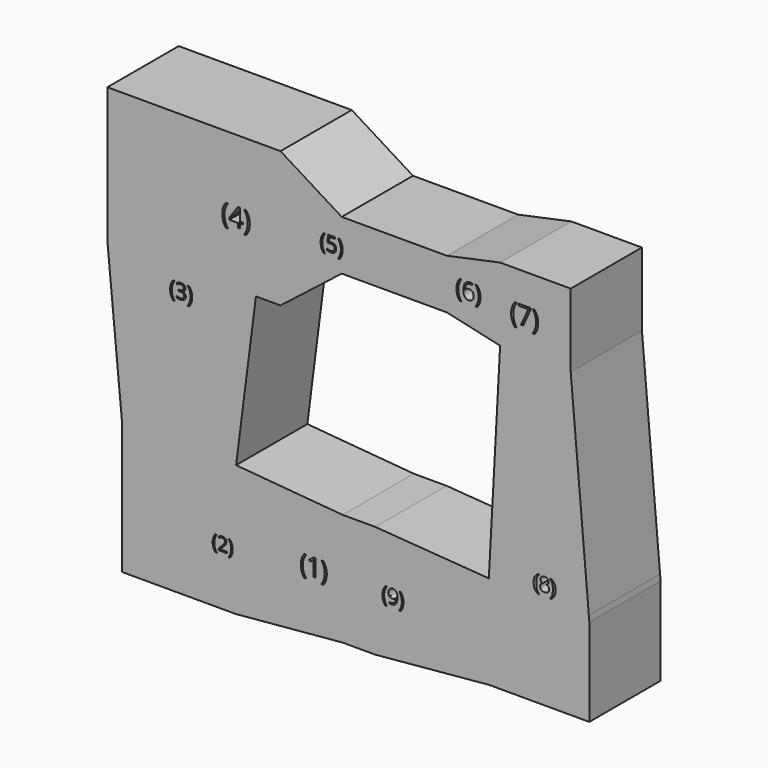
from build123d import *

# Parameters (mm, degrees)
F0_W     = 7.0054735818
F0_H     = 3.606621176
F0_H_2   = 2.8473325074
F0_H_3   = 3.0371509492
F0_H_4   = 3.4167952836
F0_H_5   = 3.4167990088
F0_H_6   = 3.0424887748
F0_H_7   = 3.4114611833
F0_H_8   = 3.2269731164
F0_H_9   = 2.668182266
F0_W_2   = 20.1211348176
F0_H_10  = 20.8804234862
F0_W_3   = 9.3167445157
F0_H_11  = 32.0711014792
F1_DEPTH = 12.7


with BuildPart() as f1:
    # F0 (on Front) → F1 (new body, symmetric)
    with BuildSketch(Plane.XZ):
        Polygon((-30.1637667992, 35.9712801874), (-72.5167479517, 35.9712801874), (-68.335942924, -8.2572624087), (-35.8229727803, -8.2572624087), align=None)
        with BuildLine():
            add(Edge.make_bspline(
                [(-54.4081610007, 28.3956593022), (-54.6265717389, 29.0386568902), (-54.6265717389, 29.777265818)],
                knots=[0, 0, 0, 1, 1, 1], degree=2))
            add(Edge.make_bspline(
                [(-54.6265717389, 29.777265818), (-54.6265717389, 30.5276562378), (-54.4068015978, 31.1819821836)],
                knots=[0, 0, 0, 1, 1, 1], degree=2))
            add(Edge.make_bspline(
                [(-54.4068015978, 31.1819821836), (-54.1870314567, 31.8363081294), (-53.7737729646, 32.3293182604)],
                knots=[0, 0, 0, 1, 1, 1], degree=2))
            Line((-53.7737729646, 32.3293182604), (-53.3152010414, 32.3293182604))
            add(Edge.make_bspline(
                [(-53.3152010414, 32.3293182604), (-53.7230219217, 31.7828382807), (-53.9282917649, 31.1285123349)],
                knots=[0, 0, 0, 1, 1, 1], degree=2))
            add(Edge.make_bspline(
                [(-53.9282917649, 31.1285123349), (-54.133561608, 30.4741863891), (-54.133561608, 29.7827034297)],
                knots=[0, 0, 0, 1, 1, 1], degree=2))
            add(Edge.make_bspline(
                [(-54.133561608, 29.7827034297), (-54.133561608, 29.1030019624), (-53.9237604217, 28.4545667627)],
                knots=[0, 0, 0, 1, 1, 1], degree=2))
            add(Edge.make_bspline(
                [(-53.9237604217, 28.4545667627), (-53.7139592355, 27.8061315629), (-53.3206386531, 27.2705268067)],
                knots=[0, 0, 0, 1, 1, 1], degree=2))
            Line((-53.3206386531, 27.2705268067), (-53.7737729646, 27.2705268067))
            add(Edge.make_bspline(
                [(-53.7737729646, 27.2705268067), (-54.1897502626, 27.7526617142), (-54.4081610007, 28.3956593022)],
                knots=[0, 0, 0, 1, 1, 1], degree=2))
        make_face(mode=Mode.SUBTRACT)
        with BuildLine():
            add(Edge.make_bspline(
                [(-50.6272083055, 32.1122669251), (-50.2927951836, 31.8363081294), (-50.2927951836, 31.3550794906)],
                knots=[0, 0, 0, 1, 1, 1], degree=2))
            add(Edge.make_bspline(
                [(-50.2927951836, 31.3550794906), (-50.2927951836, 30.9581338337), (-50.5152841306, 30.7061911565)],
                knots=[0, 0, 0, 1, 1, 1], degree=2))
            add(Edge.make_bspline(
                [(-50.5152841306, 30.7061911565), (-50.7377730775, 30.4542484793), (-51.1455939579, 30.3690592288)],
                knots=[0, 0, 0, 1, 1, 1], degree=2))
            Line((-51.1455939579, 30.3690592288), (-51.1455939579, 30.3464025132))
            add(Edge.make_bspline(
                [(-51.1455939579, 30.3464025132), (-50.6471462152, 30.2847762468), (-50.4065318958, 30.0296616295)],
                knots=[0, 0, 0, 1, 1, 1], degree=2))
            add(Edge.make_bspline(
                [(-50.4065318958, 30.0296616295), (-50.1659175764, 29.7745470121), (-50.1659175764, 29.36128852)],
                knots=[0, 0, 0, 1, 1, 1], degree=2))
            add(Edge.make_bspline(
                [(-50.1659175764, 29.36128852), (-50.1659175764, 28.7694951092), (-50.5764572627, 28.4504885539)],
                knots=[0, 0, 0, 1, 1, 1], degree=2))
            add(Edge.make_bspline(
                [(-50.5764572627, 28.4504885539), (-50.9869969489, 28.1314819986), (-51.7428249805, 28.1314819986)],
                knots=[0, 0, 0, 1, 1, 1], degree=2))
            add(Edge.make_bspline(
                [(-51.7428249805, 28.1314819986), (-52.0718004906, 28.1314819986), (-52.3450404805, 28.1813267728)],
                knots=[0, 0, 0, 1, 1, 1], degree=2))
            add(Edge.make_bspline(
                [(-52.3450404805, 28.1813267728), (-52.6182804703, 28.2311715471), (-52.8756607592, 28.3553303485)],
                knots=[0, 0, 0, 1, 1, 1], degree=2))
            Line((-52.8756607592, 28.3553303485), (-52.8756607592, 28.8030270482))
            add(Edge.make_bspline(
                [(-52.8756607592, 28.8030270482), (-52.6064989782, 28.6698055606), (-52.3019927209, 28.600476011)],
                knots=[0, 0, 0, 1, 1, 1], degree=2))
            add(Edge.make_bspline(
                [(-52.3019927209, 28.600476011), (-51.9974864635, 28.5311464613), (-51.7256058766, 28.5311464613)],
                knots=[0, 0, 0, 1, 1, 1], degree=2))
            add(Edge.make_bspline(
                [(-51.7256058766, 28.5311464613), (-50.652583827, 28.5311464613), (-50.652583827, 29.3721637435)],
                knots=[0, 0, 0, 1, 1, 1], degree=2))
            add(Edge.make_bspline(
                [(-50.652583827, 29.3721637435), (-50.652583827, 30.1261792378), (-51.8361706486, 30.1261792378)],
                knots=[0, 0, 0, 1, 1, 1], degree=2))
            Line((-51.8361706486, 30.1261792378), (-52.243991529, 30.1261792378))
            Line((-52.243991529, 30.1261792378), (-52.243991529, 30.5303750437))
            Line((-52.243991529, 30.5303750437), (-51.8307330369, 30.5303750437))
            add(Edge.make_bspline(
                [(-51.8307330369, 30.5303750437), (-51.3467855922, 30.5303750437), (-51.0635766475, 30.7442544387)],
                knots=[0, 0, 0, 1, 1, 1], degree=2))
            add(Edge.make_bspline(
                [(-51.0635766475, 30.7442544387), (-50.7803677028, 30.9581338337), (-50.7803677028, 31.3378603868)],
                knots=[0, 0, 0, 1, 1, 1], degree=2))
            add(Edge.make_bspline(
                [(-50.7803677028, 31.3378603868), (-50.7803677028, 31.6405541069), (-50.9883563518, 31.8136514139)],
                knots=[0, 0, 0, 1, 1, 1], degree=2))
            add(Edge.make_bspline(
                [(-50.9883563518, 31.8136514139), (-51.1963450008, 31.9867487209), (-51.5534148383, 31.9867487209)],
                knots=[0, 0, 0, 1, 1, 1], degree=2))
            add(Edge.make_bspline(
                [(-51.5534148383, 31.9867487209), (-51.8252954252, 31.9867487209), (-52.0659097446, 31.9128878281)],
                knots=[0, 0, 0, 1, 1, 1], degree=2))
            add(Edge.make_bspline(
                [(-52.0659097446, 31.9128878281), (-52.306524064, 31.8390269353), (-52.6155616644, 31.6405541069)],
                knots=[0, 0, 0, 1, 1, 1], degree=2))
            Line((-52.6155616644, 31.6405541069), (-52.8530040437, 31.9577481249))
            add(Edge.make_bspline(
                [(-52.8530040437, 31.9577481249), (-52.5983425606, 32.1589397592), (-52.2657419759, 32.27358274)],
                knots=[0, 0, 0, 1, 1, 1], degree=2))
            add(Edge.make_bspline(
                [(-52.2657419759, 32.27358274), (-51.9331413913, 32.3882257209), (-51.5642900617, 32.3882257209)],
                knots=[0, 0, 0, 1, 1, 1], degree=2))
            add(Edge.make_bspline(
                [(-51.5642900617, 32.3882257209), (-50.9616214274, 32.3882257209), (-50.6272083055, 32.1122669251)],
                knots=[0, 0, 0, 1, 1, 1], degree=2))
        make_face(mode=Mode.SUBTRACT)
        with BuildLine():
            add(Edge.make_bspline(
                [(-48.5600095765, 31.1779039748), (-48.3415988383, 30.5222186261), (-48.3415988383, 29.777265818)],
                knots=[0, 0, 0, 1, 1, 1], degree=2))
            add(Edge.make_bspline(
                [(-48.3415988383, 29.777265818), (-48.3415988383, 29.0323130098), (-48.5613689794, 28.3893154218)],
                knots=[0, 0, 0, 1, 1, 1], degree=2))
            add(Edge.make_bspline(
                [(-48.5613689794, 28.3893154218), (-48.7811391205, 27.7463178338), (-49.1943976126, 27.2705268067)],
                knots=[0, 0, 0, 1, 1, 1], degree=2))
            Line((-49.1943976126, 27.2705268067), (-49.6475319241, 27.2705268067))
            add(Edge.make_bspline(
                [(-49.6475319241, 27.2705268067), (-49.2542113417, 27.803412757), (-49.0444101555, 28.4532073597)],
                knots=[0, 0, 0, 1, 1, 1], degree=2))
            add(Edge.make_bspline(
                [(-49.0444101555, 28.4532073597), (-48.8346089692, 29.1030019624), (-48.8346089692, 29.7827034297)],
                knots=[0, 0, 0, 1, 1, 1], degree=2))
            add(Edge.make_bspline(
                [(-48.8346089692, 29.7827034297), (-48.8346089692, 30.4741863891), (-49.0398788123, 31.1285123349)],
                knots=[0, 0, 0, 1, 1, 1], degree=2))
            add(Edge.make_bspline(
                [(-49.0398788123, 31.1285123349), (-49.2451486554, 31.7828382807), (-49.6529695358, 32.3293182604)],
                knots=[0, 0, 0, 1, 1, 1], degree=2))
            Line((-49.6529695358, 32.3293182604), (-49.1943976126, 32.3293182604))
            add(Edge.make_bspline(
                [(-49.1943976126, 32.3293182604), (-48.7784203146, 31.8335893236), (-48.5600095765, 31.1779039748)],
                knots=[0, 0, 0, 1, 1, 1], degree=2))
        make_face(mode=Mode.SUBTRACT)
        Polygon((-30.1637667992, 74.7056555869), (-72.5167479517, 74.7056555869), (-72.5167479517, 35.9712801874), (-30.1637667992, 35.9712801874), (-30.1637667992, 39.5779013634), (-30.1637667992, 42.4252338707), (-30.1637667992, 45.46238482), (-30.1637667992, 48.8791801035), (-30.1637667992, 52.2959791124), (-30.1637667992, 55.3384678871), (-30.1637667992, 58.7499290705), (-30.1637667992, 62.1667280793), (-30.1637667992, 65.3937011957), (-30.1637667992, 68.8105002046), (-30.1637667992, 72.037473321), align=None)
        with BuildLine():
            add(Edge.make_bspline(
                [(-39.489436089, 51.7955468905), (-39.7624492438, 52.5992930868), (-39.7624492438, 53.5225533406)],
                knots=[0, 0, 0, 1, 1, 1], degree=2))
            add(Edge.make_bspline(
                [(-39.7624492438, 53.5225533406), (-39.7624492438, 54.460540445), (-39.487736837, 55.2784470747)],
                knots=[0, 0, 0, 1, 1, 1], degree=2))
            add(Edge.make_bspline(
                [(-39.487736837, 55.2784470747), (-39.2130244303, 56.0963537044), (-38.696451822, 56.7126157633)],
                knots=[0, 0, 0, 1, 1, 1], degree=2))
            Line((-38.696451822, 56.7126157633), (-38.1232374805, 56.7126157633))
            add(Edge.make_bspline(
                [(-38.1232374805, 56.7126157633), (-38.6330130807, 56.029516459), (-38.8896001328, 55.2116098293)],
                knots=[0, 0, 0, 1, 1, 1], degree=2))
            add(Edge.make_bspline(
                [(-38.8896001328, 55.2116098293), (-39.1461871849, 54.3937031996), (-39.1461871849, 53.5293503486)],
                knots=[0, 0, 0, 1, 1, 1], degree=2))
            add(Edge.make_bspline(
                [(-39.1461871849, 53.5293503486), (-39.1461871849, 52.6797243482), (-38.8839359594, 51.8691811439)],
                knots=[0, 0, 0, 1, 1, 1], degree=2))
            add(Edge.make_bspline(
                [(-38.8839359594, 51.8691811439), (-38.621684734, 51.0586379395), (-38.1300344885, 50.3891326512)],
                knots=[0, 0, 0, 1, 1, 1], degree=2))
            Line((-38.1300344885, 50.3891326512), (-38.696451822, 50.3891326512))
            add(Edge.make_bspline(
                [(-38.696451822, 50.3891326512), (-39.2164229343, 50.9918006941), (-39.489436089, 51.7955468905)],
                knots=[0, 0, 0, 1, 1, 1], degree=2))
        make_face(mode=Mode.SUBTRACT)
        Polygon((-33.9068268493, 53.2608685325), (-33.9068268493, 52.7261705696), (-34.6748887536, 52.7261705696), (-34.6748887536, 51.536694169), (-35.2379075832, 51.536694169), (-35.2379075832, 52.7261705696), (-37.7550662136, 52.7261705696), (-37.7550662136, 53.2393446738), (-35.2979478206, 56.74093663), (-34.6748887536, 56.74093663), (-34.6748887536, 53.2608685325), align=None, mode=Mode.SUBTRACT)
        with BuildLine():
            add(Edge.make_bspline(
                [(-32.1792539819, 55.2733493187), (-31.9062408271, 54.453743437), (-31.9062408271, 53.5225533406)],
                knots=[0, 0, 0, 1, 1, 1], degree=2))
            add(Edge.make_bspline(
                [(-31.9062408271, 53.5225533406), (-31.9062408271, 52.5913632442), (-32.1809532339, 51.7876170478)],
                knots=[0, 0, 0, 1, 1, 1], degree=2))
            add(Edge.make_bspline(
                [(-32.1809532339, 51.7876170478), (-32.4556656407, 50.9838708515), (-32.9722382489, 50.3891326512)],
                knots=[0, 0, 0, 1, 1, 1], degree=2))
            Line((-32.9722382489, 50.3891326512), (-33.5386555825, 50.3891326512))
            add(Edge.make_bspline(
                [(-33.5386555825, 50.3891326512), (-33.0470053369, 51.0552394355), (-32.7847541115, 51.8674818919)],
                knots=[0, 0, 0, 1, 1, 1], degree=2))
            add(Edge.make_bspline(
                [(-32.7847541115, 51.8674818919), (-32.522502886, 52.6797243482), (-32.522502886, 53.5293503486)],
                knots=[0, 0, 0, 1, 1, 1], degree=2))
            add(Edge.make_bspline(
                [(-32.522502886, 53.5293503486), (-32.522502886, 54.3937031996), (-32.7790899381, 55.2116098293)],
                knots=[0, 0, 0, 1, 1, 1], degree=2))
            add(Edge.make_bspline(
                [(-32.7790899381, 55.2116098293), (-33.0356769902, 56.029516459), (-33.5454525905, 56.7126157633)],
                knots=[0, 0, 0, 1, 1, 1], degree=2))
            Line((-33.5454525905, 56.7126157633), (-32.9722382489, 56.7126157633))
            add(Edge.make_bspline(
                [(-32.9722382489, 56.7126157633), (-32.4522671367, 56.0929552004), (-32.1792539819, 55.2733493187)],
                knots=[0, 0, 0, 1, 1, 1], degree=2))
        make_face(mode=Mode.SUBTRACT)
        with Locations((-26.6610300083, 37.7745907754)):
            Rectangle(F0_W, F0_H)
        with Locations((-26.6610300083, 41.0015676171)):
            Rectangle(F0_W, F0_H_2)
        with Locations((-26.6610300083, 43.9438093454)):
            Rectangle(F0_W, F0_H_3)
        with Locations((-26.6610300083, 47.1707824618)):
            Rectangle(F0_W, F0_H_4)
        with Locations((-26.6610300083, 50.587579608)):
            Rectangle(F0_W, F0_H_5)
        with Locations((-26.6610300083, 53.8172234998)):
            Rectangle(F0_W, F0_H_6)
        with Locations((-26.6610300083, 57.0441984788)):
            Rectangle(F0_W, F0_H_7)
        with Locations((-26.6610300083, 60.4583285749)):
            Rectangle(F0_W, F0_H_5)
        with Locations((-26.6610300083, 63.7802146375)):
            Rectangle(F0_W, F0_H_8)
        with Locations((-26.6610300083, 67.1021007001)):
            Rectangle(F0_W, F0_H_5)
        with Locations((-26.6610300083, 70.4239867628)):
            Rectangle(F0_W, F0_H_8)
        with Locations((-26.6610300083, 73.3715644539)):
            Rectangle(F0_W, F0_H_9)
        with BuildLine():
            Line((-5.6946617551, 63.8751238585), (-23.1582932174, 74.7056555869))
            Line((-23.1582932174, 74.7056555869), (-23.1582932174, 72.037473321))
            Line((-23.1582932174, 72.037473321), (-23.1582932174, 68.8105002046))
            Line((-23.1582932174, 68.8105002046), (-23.1582932174, 65.3937011957))
            Line((-23.1582932174, 65.3937011957), (-23.1582932174, 62.1667280793))
            Line((-23.1582932174, 62.1667280793), (-23.1582932174, 58.7499290705))
            Line((-23.1582932174, 58.7499290705), (-23.1582932174, 55.3384678871))
            Line((-23.1582932174, 55.3384678871), (-23.1582932174, 52.2959791124))
            Line((-23.1582932174, 52.2959791124), (-23.1582932174, 48.8791801035))
            Line((-23.1582932174, 48.8791801035), (-23.1582932174, 45.46238482))
            Line((-23.1582932174, 45.46238482), (-23.1582932174, 42.4252338707))
            Line((-23.1582932174, 42.4252338707), (-23.1582932174, 39.5779013634))
            Line((-23.1582932174, 39.5779013634), (-23.1582932174, 35.9712801874))
            Line((-23.1582932174, 35.9712801874), (-5.6946617551, 49.6384687722))
            Line((-5.6946617551, 49.6384687722), (-5.6946617551, 54.1122225139))
            add(Edge.make_bspline(
                [(-5.6946617551, 54.1122225139), (-5.9114864573, 53.5274189294), (-6.2946085915, 53.0863243669)],
                knots=[0.0729241608, 0.0729241608, 0.0729241608, 1, 1, 1], degree=2))
            Line((-6.2946085915, 53.0863243669), (-6.7477431051, 53.0863243669))
            add(Edge.make_bspline(
                [(-6.7477431051, 53.0863243669), (-6.3544223473, 53.6192105549), (-6.1446210675, 54.2690054475)],
                knots=[0, 0, 0, 1, 1, 1], degree=2))
            add(Edge.make_bspline(
                [(-6.1446210675, 54.2690054475), (-5.9348197877, 54.91880034), (-5.9348197877, 55.5985021104)],
                knots=[0, 0, 0, 1, 1, 1], degree=2))
            add(Edge.make_bspline(
                [(-5.9348197877, 55.5985021104), (-5.9348197877, 56.2899853782), (-6.1400897224, 56.9443116159)],
                knots=[0, 0, 0, 1, 1, 1], degree=2))
            add(Edge.make_bspline(
                [(-6.1400897224, 56.9443116159), (-6.345359657, 57.5986378535), (-6.7531807193, 58.1451180769)],
                knots=[0, 0, 0, 1, 1, 1], degree=2))
            Line((-6.7531807193, 58.1451180769), (-6.2946085915, 58.1451180769))
            add(Edge.make_bspline(
                [(-6.2946085915, 58.1451180769), (-5.9103361757, 57.6871725183), (-5.6946617551, 57.0927244543)],
                knots=[0, 0, 0, 0.9237817695, 0.9237817695, 0.9237817695], degree=2))
            Line((-5.6946617551, 57.0927244543), (-5.6946617551, 63.8751238585))
        make_face()
        with BuildLine():
            add(Edge.make_bspline(
                [(-11.5083743052, 54.2114573642), (-11.7267851407, 54.8544552391), (-11.7267851407, 55.5930644963)],
                knots=[0, 0, 0, 1, 1, 1], degree=2))
            add(Edge.make_bspline(
                [(-11.7267851407, 55.5930644963), (-11.7267851407, 56.3434552508), (-11.5070149016, 56.9977814885)],
                knots=[0, 0, 0, 1, 1, 1], degree=2))
            add(Edge.make_bspline(
                [(-11.5070149016, 56.9977814885), (-11.2872446625, 57.6521077261), (-10.8739859861, 58.1451180769)],
                knots=[0, 0, 0, 1, 1, 1], degree=2))
            Line((-10.8739859861, 58.1451180769), (-10.4154138583, 58.1451180769))
            add(Edge.make_bspline(
                [(-10.4154138583, 58.1451180769), (-10.8232349206, 57.5986378535), (-11.0285048553, 56.9443116159)],
                knots=[0, 0, 0, 1, 1, 1], degree=2))
            add(Edge.make_bspline(
                [(-11.0285048553, 56.9443116159), (-11.2337747899, 56.2899853782), (-11.2337747899, 55.5985021104)],
                knots=[0, 0, 0, 1, 1, 1], degree=2))
            add(Edge.make_bspline(
                [(-11.2337747899, 55.5985021104), (-11.2337747899, 54.91880034), (-11.0239735101, 54.270364851)],
                knots=[0, 0, 0, 1, 1, 1], degree=2))
            add(Edge.make_bspline(
                [(-11.0239735101, 54.270364851), (-10.8141722303, 53.621929362), (-10.4208514725, 53.0863243669)],
                knots=[0, 0, 0, 1, 1, 1], degree=2))
            Line((-10.4208514725, 53.0863243669), (-10.8739859861, 53.0863243669))
            add(Edge.make_bspline(
                [(-10.8739859861, 53.0863243669), (-11.2899634696, 53.5684594894), (-11.5083743052, 54.2114573642)],
                knots=[0, 0, 0, 1, 1, 1], degree=2))
        make_face(mode=Mode.SUBTRACT)
        with BuildLine():
            add(Edge.make_bspline(
                [(-9.3133907212, 56.4685203766), (-8.9880401404, 56.5337717465), (-8.6645020977, 56.5337717465)],
                knots=[0, 0, 0, 1, 1, 1], degree=2))
            add(Edge.make_bspline(
                [(-8.6645020977, 56.5337717465), (-8.0101758601, 56.5337717465), (-7.6349804828, 56.2093274348)],
                knots=[0, 0, 0, 1, 1, 1], degree=2))
            add(Edge.make_bspline(
                [(-7.6349804828, 56.2093274348), (-7.2597851055, 55.884883123), (-7.2597851055, 55.3211837881)],
                knots=[0, 0, 0, 1, 1, 1], degree=2))
            add(Edge.make_bspline(
                [(-7.2597851055, 55.3211837881), (-7.2597851055, 54.6786390478), (-7.6689655713, 54.3129594953)],
                knots=[0, 0, 0, 1, 1, 1], degree=2))
            add(Edge.make_bspline(
                [(-7.6689655713, 54.3129594953), (-8.0781460371, 53.9472799428), (-8.7977236447, 53.9472799428)],
                knots=[0, 0, 0, 1, 1, 1], degree=2))
            add(Edge.make_bspline(
                [(-8.7977236447, 53.9472799428), (-9.4973633337, 53.9472799428), (-9.8653085588, 54.1711283925)],
                knots=[0, 0, 0, 1, 1, 1], degree=2))
            Line((-9.8653085588, 54.1711283925), (-9.8653085588, 54.6242629061))
            add(Edge.make_bspline(
                [(-9.8653085588, 54.6242629061), (-9.6677419109, 54.4973852423), (-9.373204477, 54.4248837202)],
                knots=[0, 0, 0, 1, 1, 1], degree=2))
            add(Edge.make_bspline(
                [(-9.373204477, 54.4248837202), (-9.0786670432, 54.352382198), (-8.7922860306, 54.352382198)],
                knots=[0, 0, 0, 1, 1, 1], degree=2))
            add(Edge.make_bspline(
                [(-8.7922860306, 54.352382198), (-8.2938380656, 54.352382198), (-8.0178791468, 54.5875590105)],
                knots=[0, 0, 0, 1, 1, 1], degree=2))
            add(Edge.make_bspline(
                [(-8.0178791468, 54.5875590105), (-7.741920228, 54.8227358231), (-7.741920228, 55.2677139155)],
                knots=[0, 0, 0, 1, 1, 1], degree=2))
            add(Edge.make_bspline(
                [(-7.741920228, 55.2677139155), (-7.741920228, 56.1341071055), (-8.8031612589, 56.1341071055)],
                knots=[0, 0, 0, 1, 1, 1], degree=2))
            add(Edge.make_bspline(
                [(-8.8031612589, 56.1341071055), (-9.07232316, 56.1341071055), (-9.5227388665, 56.051636624)],
                knots=[0, 0, 0, 1, 1, 1], degree=2))
            Line((-9.5227388665, 56.051636624), (-9.7665252348, 56.2075148967))
            Line((-9.7665252348, 56.2075148967), (-9.6106469621, 58.1451180769))
            Line((-9.6106469621, 58.1451180769), (-7.5516037323, 58.1451180769))
            Line((-7.5516037323, 58.1451180769), (-7.5516037323, 57.7119214819))
            Line((-7.5516037323, 57.7119214819), (-9.2082635141, 57.7119214819))
            Line((-9.2082635141, 57.7119214819), (-9.3133907212, 56.4685203766))
        make_face(mode=Mode.SUBTRACT)
        with BuildLine():
            Line((24.2972243577, 63.8751238585), (-5.6946617551, 63.8751238585))
            Line((-5.6946617551, 63.8751238585), (-5.6946617551, 57.0927244543))
            add(Edge.make_bspline(
                [(-5.6946617551, 57.0927244543), (-5.6768671599, 57.0436784772), (-5.6602202725, 56.9937032778)],
                knots=[0.9237817695, 0.9237817695, 0.9237817695, 1, 1, 1], degree=2))
            add(Edge.make_bspline(
                [(-5.6602202725, 56.9937032778), (-5.4418094369, 56.3380176366), (-5.4418094369, 55.5930644963)],
                knots=[0, 0, 0, 1, 1, 1], degree=2))
            add(Edge.make_bspline(
                [(-5.4418094369, 55.5930644963), (-5.4418094369, 54.8481113559), (-5.661579676, 54.2051134811)],
                knots=[0, 0, 0, 1, 1, 1], degree=2))
            add(Edge.make_bspline(
                [(-5.661579676, 54.2051134811), (-5.6776062363, 54.1582234006), (-5.6946617551, 54.1122225139)],
                knots=[0, 0, 0, 0.0729241608, 0.0729241608, 0.0729241608], degree=2))
            Line((-5.6946617551, 54.1122225139), (-5.6946617551, 49.6384687722))
            Line((-5.6946617551, 49.6384687722), (24.2972243577, 49.6384687722))
            Line((24.2972243577, 49.6384687722), (24.2972243577, 63.8751238585))
        make_face()
        Polygon((39.4829921424, 67.1020969748), (24.2972243577, 63.8751238585), (24.2972243577, 49.6384687722), (39.4829921424, 46.2216734886), align=None)
        with BuildLine():
            add(Edge.make_bspline(
                [(27.2562728553, 54.9895752528), (27.0180066841, 55.6910269063), (27.0180066841, 56.4967818007)],
                knots=[0, 0, 0, 1, 1, 1], degree=2))
            add(Edge.make_bspline(
                [(27.0180066841, 56.4967818007), (27.0180066841, 57.3153892272), (27.2577558398, 58.0291990846)],
                knots=[0, 0, 0, 1, 1, 1], degree=2))
            add(Edge.make_bspline(
                [(27.2577558398, 58.0291990846), (27.4975049955, 58.7430089419), (27.9483322738, 59.2808379758)],
                knots=[0, 0, 0, 1, 1, 1], degree=2))
            Line((27.9483322738, 59.2808379758), (28.4485923678, 59.2808379758))
            add(Edge.make_bspline(
                [(28.4485923678, 59.2808379758), (28.0036970273, 58.6846782195), (27.7797663726, 57.9708683621)],
                knots=[0, 0, 0, 1, 1, 1], degree=2))
            add(Edge.make_bspline(
                [(27.7797663726, 57.9708683621), (27.5558357179, 57.2570585047), (27.5558357179, 56.5027137386)],
                knots=[0, 0, 0, 1, 1, 1], degree=2))
            add(Edge.make_bspline(
                [(27.5558357179, 56.5027137386), (27.5558357179, 55.7612215044), (27.7847096541, 55.0538379131)],
                knots=[0, 0, 0, 1, 1, 1], degree=2))
            add(Edge.make_bspline(
                [(27.7847096541, 55.0538379131), (28.0135835904, 54.3464543217), (28.4426604299, 53.7621584412)],
                knots=[0, 0, 0, 1, 1, 1], degree=2))
            Line((28.4426604299, 53.7621584412), (27.9483322738, 53.7621584412))
            add(Edge.make_bspline(
                [(27.9483322738, 53.7621584412), (27.4945390265, 54.2881235993), (27.2562728553, 54.9895752528)],
                knots=[0, 0, 0, 1, 1, 1], degree=2))
        make_face(mode=Mode.SUBTRACT)
        with BuildLine():
            add(Edge.make_bspline(
                [(29.4100606314, 55.2283357522), (28.9992739337, 55.7552895666), (28.9992739337, 56.6945130631)],
                knots=[0, 0, 0, 1, 1, 1], degree=2))
            add(Edge.make_bspline(
                [(28.9992739337, 56.6945130631), (28.9992739337, 58.0262331156), (29.5168355131, 58.6856668758)],
                knots=[0, 0, 0, 1, 1, 1], degree=2))
            add(Edge.make_bspline(
                [(29.5168355131, 58.6856668758), (30.0343970925, 59.3451006361), (31.0477698125, 59.3451006361)],
                knots=[0, 0, 0, 1, 1, 1], degree=2))
            add(Edge.make_bspline(
                [(31.0477698125, 59.3451006361), (31.3967654907, 59.3451006361), (31.597462722, 59.2867699136)],
                knots=[0, 0, 0, 1, 1, 1], degree=2))
            Line((31.597462722, 59.2867699136), (31.597462722, 58.8448405421))
            add(Edge.make_bspline(
                [(31.597462722, 58.8448405421), (31.3591965508, 58.9219557345), (31.0537017504, 58.9219557345)],
                knots=[0, 0, 0, 1, 1, 1], degree=2))
            add(Edge.make_bspline(
                [(31.0537017504, 58.9219557345), (30.3270393609, 58.9219557345), (29.9439350399, 58.4696454716)],
                knots=[0, 0, 0, 1, 1, 1], degree=2))
            add(Edge.make_bspline(
                [(29.9439350399, 58.4696454716), (29.560830719, 58.0173352088), (29.5242504354, 57.0464747103)],
                knots=[0, 0, 0, 1, 1, 1], degree=2))
            Line((29.5242504354, 57.0464747103), (29.560830719, 57.0464747103))
            add(Edge.make_bspline(
                [(29.560830719, 57.0464747103), (29.9009284904, 57.5783718062), (30.6364887866, 57.5783718062)],
                knots=[0, 0, 0, 1, 1, 1], degree=2))
            add(Edge.make_bspline(
                [(30.6364887866, 57.5783718062), (31.2455010749, 57.5783718062), (31.5959797376, 57.2105916581)],
                knots=[0, 0, 0, 1, 1, 1], degree=2))
            add(Edge.make_bspline(
                [(31.5959797376, 57.2105916581), (31.9464584002, 56.8428115099), (31.9464584002, 56.2130374391)],
                knots=[0, 0, 0, 1, 1, 1], degree=2))
            add(Edge.make_bspline(
                [(31.9464584002, 56.2130374391), (31.9464584002, 55.5081254885), (31.5618710948, 55.1047537131)],
                knots=[0, 0, 0, 1, 1, 1], degree=2))
            add(Edge.make_bspline(
                [(31.5618710948, 55.1047537131), (31.1772837894, 54.7013819378), (30.5218046544, 54.7013819378)],
                knots=[0, 0, 0, 1, 1, 1], degree=2))
            add(Edge.make_bspline(
                [(30.5218046544, 54.7013819378), (29.8208473291, 54.7013819378), (29.4100606314, 55.2283357522)],
                knots=[0, 0, 0, 1, 1, 1], degree=2))
        make_face(mode=Mode.SUBTRACT)
        with BuildLine():
            add(Edge.make_bspline(
                [(33.6360720378, 58.0247501312), (33.874338209, 57.3094572893), (33.874338209, 56.4967818007)],
                knots=[0, 0, 0, 1, 1, 1], degree=2))
            add(Edge.make_bspline(
                [(33.874338209, 56.4967818007), (33.874338209, 55.6841063121), (33.6345890533, 54.9826546586)],
                knots=[0, 0, 0, 1, 1, 1], degree=2))
            add(Edge.make_bspline(
                [(33.6345890533, 54.9826546586), (33.3948398976, 54.2812030051), (32.9440126192, 53.7621584412)],
                knots=[0, 0, 0, 1, 1, 1], degree=2))
            Line((32.9440126192, 53.7621584412), (32.4496844631, 53.7621584412))
            add(Edge.make_bspline(
                [(32.4496844631, 53.7621584412), (32.8787613026, 54.3434883528), (33.1076352389, 55.0523549286)],
                knots=[0, 0, 0, 1, 1, 1], degree=2))
            add(Edge.make_bspline(
                [(33.1076352389, 55.0523549286), (33.3365091752, 55.7612215044), (33.3365091752, 56.5027137386)],
                knots=[0, 0, 0, 1, 1, 1], degree=2))
            add(Edge.make_bspline(
                [(33.3365091752, 56.5027137386), (33.3365091752, 57.2570585047), (33.1125785205, 57.9708683621)],
                knots=[0, 0, 0, 1, 1, 1], degree=2))
            add(Edge.make_bspline(
                [(33.1125785205, 57.9708683621), (32.8886478657, 58.6846782195), (32.4437525253, 59.2808379758)],
                knots=[0, 0, 0, 1, 1, 1], degree=2))
            Line((32.4437525253, 59.2808379758), (32.9440126192, 59.2808379758))
            add(Edge.make_bspline(
                [(32.9440126192, 59.2808379758), (33.3978058665, 58.740042973), (33.6360720378, 58.0247501312)],
                knots=[0, 0, 0, 1, 1, 1], degree=2))
        make_face(mode=Mode.SUBTRACT)
        with Locations((49.5435595512, 56.6618852317)):
            Rectangle(F0_W_2, F0_H_10)
        with BuildLine():
            add(Edge.make_bspline(
                [(42.8831042389, 53.6890552458), (42.6150543822, 54.4781895749), (42.6150543822, 55.3846652312)],
                knots=[0, 0, 0, 1, 1, 1], degree=2))
            add(Edge.make_bspline(
                [(42.6150543822, 55.3846652312), (42.6150543822, 56.3056000085), (42.884772599, 57.1086373384)],
                knots=[0, 0, 0, 1, 1, 1], degree=2))
            add(Edge.make_bspline(
                [(42.884772599, 57.1086373384), (43.1544908157, 57.9116746683), (43.6616722873, 58.5167332659)],
                knots=[0, 0, 0, 1, 1, 1], degree=2))
            Line((43.6616722873, 58.5167332659), (44.2244657623, 58.5167332659))
            add(Edge.make_bspline(
                [(44.2244657623, 58.5167332659), (43.7239577311, 57.8460525042), (43.4720353555, 57.0430151743)],
                knots=[0, 0, 0, 1, 1, 1], degree=2))
            add(Edge.make_bspline(
                [(43.4720353555, 57.0430151743), (43.2201129798, 56.2399778444), (43.2201129798, 55.3913386716)],
                knots=[0, 0, 0, 1, 1, 1], degree=2))
            add(Edge.make_bspline(
                [(43.2201129798, 55.3913386716), (43.2201129798, 54.5571586198), (43.4775965558, 53.7613508503)],
                knots=[0, 0, 0, 1, 1, 1], degree=2))
            add(Edge.make_bspline(
                [(43.4775965558, 53.7613508503), (43.7350801318, 52.9655430809), (44.2177923218, 52.3082092)],
                knots=[0, 0, 0, 1, 1, 1], degree=2))
            Line((44.2177923218, 52.3082092), (43.6616722873, 52.3082092))
            add(Edge.make_bspline(
                [(43.6616722873, 52.3082092), (43.1511540955, 52.8999209168), (42.8831042389, 53.6890552458)],
                knots=[0, 0, 0, 1, 1, 1], degree=2))
        make_face(mode=Mode.SUBTRACT)
        Polygon((46.0674475568, 53.43490839), (45.4279095171, 53.43490839), (47.5333799679, 57.9850825129), (44.7639021958, 57.9850825129), (44.7639021958, 58.5167332659), (48.1451120059, 58.5167332659), (48.1451120059, 58.0540413971), align=None, mode=Mode.SUBTRACT)
        with BuildLine():
            add(Edge.make_bspline(
                [(50.060389405, 57.1036322581), (50.3284392616, 56.2989265681), (50.3284392616, 55.3846652312)],
                knots=[0, 0, 0, 1, 1, 1], degree=2))
            add(Edge.make_bspline(
                [(50.3284392616, 55.3846652312), (50.3284392616, 54.4704038944), (50.0587210449, 53.6812695654)],
                knots=[0, 0, 0, 1, 1, 1], degree=2))
            add(Edge.make_bspline(
                [(50.0587210449, 53.6812695654), (49.7890028281, 52.8921352363), (49.2818213566, 52.3082092)],
                knots=[0, 0, 0, 1, 1, 1], degree=2))
            Line((49.2818213566, 52.3082092), (48.725701322, 52.3082092))
            add(Edge.make_bspline(
                [(48.725701322, 52.3082092), (49.208413512, 52.9622063607), (49.465897088, 53.7596824902)],
                knots=[0, 0, 0, 1, 1, 1], degree=2))
            add(Edge.make_bspline(
                [(49.465897088, 53.7596824902), (49.723380664, 54.5571586198), (49.723380664, 55.3913386716)],
                knots=[0, 0, 0, 1, 1, 1], degree=2))
            add(Edge.make_bspline(
                [(49.723380664, 55.3913386716), (49.723380664, 56.2399778444), (49.4714582884, 57.0430151743)],
                knots=[0, 0, 0, 1, 1, 1], degree=2))
            add(Edge.make_bspline(
                [(49.4714582884, 57.0430151743), (49.2195359127, 57.8460525042), (48.7190278816, 58.5167332659)],
                knots=[0, 0, 0, 1, 1, 1], degree=2))
            Line((48.7190278816, 58.5167332659), (49.2818213566, 58.5167332659))
            add(Edge.make_bspline(
                [(49.2818213566, 58.5167332659), (49.7923395483, 57.9083379481), (50.060389405, 57.1036322581)],
                knots=[0, 0, 0, 1, 1, 1], degree=2))
        make_face(mode=Mode.SUBTRACT)
        Polygon((59.60412696, 46.2216734886), (39.4829921424, 46.2216734886), (36.2560115755, -13.2345753504), (64.7742343731, -13.2345753504), align=None)
        with BuildLine():
            add(Edge.make_bspline(
                [(49.8858438735, -9.0060435969), (49.8119829972, -9.4170363257), (49.8119829972, -10.0849561519)],
                knots=[0, 0, 0, 1, 1, 1], degree=2))
            add(Edge.make_bspline(
                [(49.8119829972, -10.0849561519), (49.8119829972, -10.7565010518), (49.8844844709, -11.1670406465)],
                knots=[0, 0, 0, 1, 1, 1], degree=2))
            add(Edge.make_bspline(
                [(49.8844844709, -11.1670406465), (49.9569859445, -11.5775802412), (50.1142235156, -11.889336578)],
                knots=[0, 0, 0, 1, 1, 1], degree=2))
            add(Edge.make_bspline(
                [(50.1142235156, -11.889336578), (50.2714610866, -12.2010929147), (50.5288413181, -12.3959406252)],
                knots=[0, 0, 0, 1, 1, 1], degree=2))
            Line((50.5288413181, -12.3959406252), (50.5288413181, -12.7194784515))
            add(Edge.make_bspline(
                [(50.5288413181, -12.7194784515), (49.9678611656, -12.421316141), (49.6520266209, -12.0687777253)],
                knots=[0, 0, 0, 1, 1, 1], degree=2))
            add(Edge.make_bspline(
                [(49.6520266209, -12.0687777253), (49.3361920762, -11.7162393096), (49.1875640552, -11.239088986)],
                knots=[0, 0, 0, 1, 1, 1], degree=2))
            add(Edge.make_bspline(
                [(49.1875640552, -11.239088986), (49.0389360342, -10.7619386624), (49.0389360342, -10.0822373467)],
                knots=[0, 0, 0, 1, 1, 1], degree=2))
            add(Edge.make_bspline(
                [(49.0389360342, -10.0822373467), (49.0389360342, -9.4079736415), (49.1875640552, -8.9321827206)],
                knots=[0, 0, 0, 1, 1, 1], degree=2))
            add(Edge.make_bspline(
                [(49.1875640552, -8.9321827206), (49.3361920762, -8.4563917996), (49.6520266209, -8.1052127865)],
                knots=[0, 0, 0, 1, 1, 1], degree=2))
            add(Edge.make_bspline(
                [(49.6520266209, -8.1052127865), (49.9678611656, -7.7540337734), (50.5288413181, -7.4594965366)],
                knots=[0, 0, 0, 1, 1, 1], degree=2))
            Line((50.5288413181, -7.4594965366), (50.5288413181, -7.7830343628))
            add(Edge.make_bspline(
                [(50.5288413181, -7.7830343628), (50.2714610866, -7.9778820733), (50.1155829182, -8.2864664707)],
                knots=[0, 0, 0, 1, 1, 1], degree=2))
            add(Edge.make_bspline(
                [(50.1155829182, -8.2864664707), (49.9597047498, -8.595050868), (49.8858438735, -9.0060435969)],
                knots=[0, 0, 0, 1, 1, 1], degree=2))
        make_face(mode=Mode.SUBTRACT)
        with BuildLine():
            add(Edge.make_bspline(
                [(54.6818163569, -12.06605892), (54.3659818122, -12.4185973358), (53.8022828544, -12.7194784515)],
                knots=[0, 0, 0, 1, 1, 1], degree=2))
            Line((53.8022828544, -12.7194784515), (53.8022828544, -12.3959406252))
            add(Edge.make_bspline(
                [(53.8022828544, -12.3959406252), (54.0605693544, -12.1983741095), (54.2178069254, -11.8866177727)],
                knots=[0, 0, 0, 1, 1, 1], degree=2))
            add(Edge.make_bspline(
                [(54.2178069254, -11.8866177727), (54.3750444964, -11.5748614359), (54.4470928359, -11.1597904991)],
                knots=[0, 0, 0, 1, 1, 1], degree=2))
            add(Edge.make_bspline(
                [(54.4470928359, -11.1597904991), (54.5191411754, -10.7447195624), (54.5191411754, -10.0849561519)],
                knots=[0, 0, 0, 1, 1, 1], degree=2))
            add(Edge.make_bspline(
                [(54.5191411754, -10.0849561519), (54.5191411754, -9.4143175205), (54.4452802991, -9.0033247916)],
                knots=[0, 0, 0, 1, 1, 1], degree=2))
            add(Edge.make_bspline(
                [(54.4452802991, -9.0033247916), (54.3714194228, -8.5923320627), (54.2159943886, -8.2864664707)],
                knots=[0, 0, 0, 1, 1, 1], degree=2))
            add(Edge.make_bspline(
                [(54.2159943886, -8.2864664707), (54.0605693544, -7.9806008786), (53.8022828544, -7.7830343628)],
                knots=[0, 0, 0, 1, 1, 1], degree=2))
            Line((53.8022828544, -7.7830343628), (53.8022828544, -7.4594965366))
            add(Edge.make_bspline(
                [(53.8022828544, -7.4594965366), (54.3687006175, -7.7630964576), (54.6831757595, -8.1129160681)],
                knots=[0, 0, 0, 1, 1, 1], degree=2))
            add(Edge.make_bspline(
                [(54.6831757595, -8.1129160681), (54.9976509016, -8.4627356785), (55.14491952, -8.9367140627)],
                knots=[0, 0, 0, 1, 1, 1], degree=2))
            add(Edge.make_bspline(
                [(55.14491952, -8.9367140627), (55.2921881384, -9.4106924468), (55.2921881384, -10.0822373467)],
                knots=[0, 0, 0, 1, 1, 1], degree=2))
            add(Edge.make_bspline(
                [(55.2921881384, -10.0822373467), (55.2921881384, -10.7592198571), (55.14491952, -11.2363701807)],
                knots=[0, 0, 0, 1, 1, 1], degree=2))
            add(Edge.make_bspline(
                [(55.14491952, -11.2363701807), (54.9976509016, -11.7135205043), (54.6818163569, -12.06605892)],
                knots=[0, 0, 0, 1, 1, 1], degree=2))
        make_face(mode=Mode.SUBTRACT)
        with BuildLine():
            add(Edge.make_bspline(
                [(53.028329623, -7.8917865734), (53.3355546177, -8.1564169523), (53.3355546177, -8.6213326522)],
                knots=[0, 0, 0, 1, 1, 1], degree=2))
            add(Edge.make_bspline(
                [(53.3355546177, -8.6213326522), (53.3355546177, -8.9321827206), (53.1823952545, -9.1519528126)],
                knots=[0, 0, 0, 1, 1, 1], degree=2))
            add(Edge.make_bspline(
                [(53.1823952545, -9.1519528126), (53.0292358914, -9.3717229047), (52.7519177546, -9.4705061626)],
                knots=[0, 0, 0, 1, 1, 1], degree=2))
            add(Edge.make_bspline(
                [(52.7519177546, -9.4705061626), (53.0772681177, -9.591946131), (53.2503653861, -9.8470606915)],
                knots=[0, 0, 0, 1, 1, 1], degree=2))
            add(Edge.make_bspline(
                [(53.2503653861, -9.8470606915), (53.4234626545, -10.1021752519), (53.4234626545, -10.4592450098)],
                knots=[0, 0, 0, 1, 1, 1], degree=2))
            add(Edge.make_bspline(
                [(53.4234626545, -10.4592450098), (53.4234626545, -10.9966621834), (53.1130657203, -11.2689958438)],
                knots=[0, 0, 0, 1, 1, 1], degree=2))
            add(Edge.make_bspline(
                [(53.1130657203, -11.2689958438), (52.8026687862, -11.5413295043), (52.1483429863, -11.5413295043)],
                knots=[0, 0, 0, 1, 1, 1], degree=2))
            add(Edge.make_bspline(
                [(52.1483429863, -11.5413295043), (50.9085677865, -11.5413295043), (50.9085677865, -10.4592450098)],
                knots=[0, 0, 0, 1, 1, 1], degree=2))
            add(Edge.make_bspline(
                [(50.9085677865, -10.4592450098), (50.9085677865, -10.0967376414), (51.0839307259, -9.8416230809)],
                knots=[0, 0, 0, 1, 1, 1], degree=2))
            add(Edge.make_bspline(
                [(51.0839307259, -9.8416230809), (51.2592936654, -9.5865085204), (51.5710500022, -9.4705061626)],
                knots=[0, 0, 0, 1, 1, 1], degree=2))
            add(Edge.make_bspline(
                [(51.5710500022, -9.4705061626), (51.2964506706, -9.3653790257), (51.1460101128, -9.1474214705)],
                knots=[0, 0, 0, 1, 1, 1], degree=2))
            add(Edge.make_bspline(
                [(51.1460101128, -9.1474214705), (50.9955695549, -8.9294639153), (50.9955695549, -8.612269968)],
                knots=[0, 0, 0, 1, 1, 1], degree=2))
            add(Edge.make_bspline(
                [(50.9955695549, -8.612269968), (50.9955695549, -8.1482605365), (51.3032476838, -7.8877083655)],
                knots=[0, 0, 0, 1, 1, 1], degree=2))
            add(Edge.make_bspline(
                [(51.3032476838, -7.8877083655), (51.6109258127, -7.6271561945), (52.1709996968, -7.6271561945)],
                knots=[0, 0, 0, 1, 1, 1], degree=2))
            add(Edge.make_bspline(
                [(52.1709996968, -7.6271561945), (52.7211046283, -7.6271561945), (53.028329623, -7.8917865734)],
                knots=[0, 0, 0, 1, 1, 1], degree=2))
        make_face(mode=Mode.SUBTRACT)
        Polygon((64.7742343731, -13.2345753504), (36.2560115755, -13.2345753504), (36.2560115755, -39.957549423), (64.9191439152, -39.957549423), (64.9191439152, -14.9010354653), align=None)
        Polygon((36.2560115755, -13.2345753504), (3.8791268598, -10.85015852), (3.8791268598, -42.9212599993), (36.2560115755, -39.957549423), align=None)
        with BuildLine():
            add(Edge.make_bspline(
                [(6.1246047509, -28.5603738826), (5.916121778, -27.9466034707), (5.916121778, -27.241567691)],
                knots=[0, 0, 0, 1, 1, 1], degree=2))
            add(Edge.make_bspline(
                [(5.916121778, -27.241567691), (5.916121778, -26.5252859418), (6.1259023627, -25.9007020977)],
                knots=[0, 0, 0, 1, 1, 1], degree=2))
            add(Edge.make_bspline(
                [(6.1259023627, -25.9007020977), (6.3356829475, -25.2761182536), (6.7301569543, -24.8055176841)],
                knots=[0, 0, 0, 1, 1, 1], degree=2))
            Line((6.7301569543, -24.8055176841), (7.1678846899, -24.8055176841))
            add(Edge.make_bspline(
                [(7.1678846899, -24.8055176841), (6.7786011306, -25.3271576536), (6.582661739, -25.9517414977)],
                knots=[0, 0, 0, 1, 1, 1], degree=2))
            add(Edge.make_bspline(
                [(6.582661739, -25.9517414977), (6.3867223475, -26.5763253418), (6.3867223475, -27.2363772436)],
                knots=[0, 0, 0, 1, 1, 1], degree=2))
            add(Edge.make_bspline(
                [(6.3867223475, -27.2363772436), (6.3867223475, -27.8851831758), (6.5869871119, -28.5041440351)],
                knots=[0, 0, 0, 1, 1, 1], degree=2))
            add(Edge.make_bspline(
                [(6.5869871119, -28.5041440351), (6.7872518763, -29.1231048945), (7.1626942424, -29.6343639691)],
                knots=[0, 0, 0, 1, 1, 1], degree=2))
            Line((7.1626942424, -29.6343639691), (6.7301569543, -29.6343639691))
            add(Edge.make_bspline(
                [(6.7301569543, -29.6343639691), (6.3330877238, -29.1741442945), (6.1246047509, -28.5603738826)],
                knots=[0, 0, 0, 1, 1, 1], degree=2))
        make_face(mode=Mode.SUBTRACT)
        with BuildLine():
            add(Edge.make_bspline(
                [(11.7069309919, -25.9045949333), (11.9154139647, -26.5304763893), (11.9154139647, -27.241567691)],
                knots=[0, 0, 0, 1, 1, 1], degree=2))
            add(Edge.make_bspline(
                [(11.9154139647, -27.241567691), (11.9154139647, -27.9526589927), (11.70563338, -28.5664294046)],
                knots=[0, 0, 0, 1, 1, 1], degree=2))
            add(Edge.make_bspline(
                [(11.70563338, -28.5664294046), (11.4958527952, -29.1801998165), (11.1013787884, -29.6343639691)],
                knots=[0, 0, 0, 1, 1, 1], degree=2))
            Line((11.1013787884, -29.6343639691), (10.6688415003, -29.6343639691))
            add(Edge.make_bspline(
                [(10.6688415003, -29.6343639691), (11.0442838664, -29.1257001182), (11.2445486308, -28.505441647)],
                knots=[0, 0, 0, 1, 1, 1], degree=2))
            add(Edge.make_bspline(
                [(11.2445486308, -28.505441647), (11.4448133952, -27.8851831758), (11.4448133952, -27.2363772436)],
                knots=[0, 0, 0, 1, 1, 1], degree=2))
            add(Edge.make_bspline(
                [(11.4448133952, -27.2363772436), (11.4448133952, -26.5763253418), (11.2488740037, -25.9517414977)],
                knots=[0, 0, 0, 1, 1, 1], degree=2))
            add(Edge.make_bspline(
                [(11.2488740037, -25.9517414977), (11.0529346122, -25.3271576536), (10.6636510528, -24.8055176841)],
                knots=[0, 0, 0, 1, 1, 1], degree=2))
            Line((10.6636510528, -24.8055176841), (11.1013787884, -24.8055176841))
            add(Edge.make_bspline(
                [(11.1013787884, -24.8055176841), (11.498448019, -25.2787134773), (11.7069309919, -25.9045949333)],
                knots=[0, 0, 0, 1, 1, 1], degree=2))
        make_face(mode=Mode.SUBTRACT)
        with BuildLine():
            add(Edge.make_bspline(
                [(10.039499746, -25.5585651028), (10.2017012291, -25.9543367214), (10.2017012291, -26.4924131079)],
                knots=[0, 0, 0, 1, 1, 1], degree=2))
            add(Edge.make_bspline(
                [(10.2017012291, -26.4924131079), (10.2017012291, -28.8125431216), (8.4066714832, -28.8125431216)],
                knots=[0, 0, 0, 1, 1, 1], degree=2))
            add(Edge.make_bspline(
                [(8.4066714832, -28.8125431216), (8.092649412, -28.8125431216), (7.9092536018, -28.7580434233)],
                knots=[0, 0, 0, 1, 1, 1], degree=2))
            Line((7.9092536018, -28.7580434233), (7.9092536018, -28.3713550877))
            add(Edge.make_bspline(
                [(7.9092536018, -28.3713550877), (8.1255222459, -28.4414261284), (8.4006159612, -28.4414261284)],
                knots=[0, 0, 0, 1, 1, 1], degree=2))
            add(Edge.make_bspline(
                [(8.4006159612, -28.4414261284), (9.0494218934, -28.4414261284), (9.3807454561, -28.040031525)],
                knots=[0, 0, 0, 1, 1, 1], degree=2))
            add(Edge.make_bspline(
                [(9.3807454561, -28.040031525), (9.7120690189, -27.6386369215), (9.7414815545, -26.8090304028)],
                knots=[0, 0, 0, 1, 1, 1], degree=2))
            Line((9.7414815545, -26.8090304028), (9.7094737951, -26.8090304028))
            add(Edge.make_bspline(
                [(9.7094737951, -26.8090304028), (9.560680968, -27.0330847181), (9.314567251, -27.1507348605)],
                knots=[0, 0, 0, 1, 1, 1], degree=2))
            add(Edge.make_bspline(
                [(9.314567251, -27.1507348605), (9.0684535341, -27.2683850029), (8.7604869849, -27.2683850029)],
                knots=[0, 0, 0, 1, 1, 1], degree=2))
            add(Edge.make_bspline(
                [(8.7604869849, -27.2683850029), (8.2362517917, -27.2683850029), (7.9278527052, -26.954795469)],
                knots=[0, 0, 0, 1, 1, 1], degree=2))
            add(Edge.make_bspline(
                [(7.9278527052, -26.954795469), (7.6194536187, -26.641205935), (7.6194536187, -26.0789074604)],
                knots=[0, 0, 0, 1, 1, 1], degree=2))
            add(Edge.make_bspline(
                [(7.6194536187, -26.0789074604), (7.6194536187, -25.4629743621), (7.9641858374, -25.1061310994)],
                knots=[0, 0, 0, 1, 1, 1], degree=2))
            add(Edge.make_bspline(
                [(7.9641858374, -25.1061310994), (8.3089180561, -24.7492878366), (8.8712165307, -24.7492878366)],
                knots=[0, 0, 0, 1, 1, 1], degree=2))
            add(Edge.make_bspline(
                [(8.8712165307, -24.7492878366), (9.2743412832, -24.7492878366), (9.5758197731, -24.9560406604)],
                knots=[0, 0, 0, 1, 1, 1], degree=2))
            add(Edge.make_bspline(
                [(9.5758197731, -24.9560406604), (9.8772982629, -25.1627934841), (10.039499746, -25.5585651028)],
                knots=[0, 0, 0, 1, 1, 1], degree=2))
        make_face(mode=Mode.SUBTRACT)
        with Locations((-0.779245398, -26.8857092597)):
            Rectangle(F0_W_3, F0_H_11)
        Polygon((-5.4376176558, -10.85015852), (-35.8229727803, -8.2572624087), (-35.8229727803, -45.6474198521), (-5.4376176558, -42.9212599993), align=None)
        with BuildLine():
            add(Edge.make_bspline(
                [(-17.1211440942, -28.8929522483), (-17.379265796, -28.1330462425), (-17.379265796, -27.260145052)],
                knots=[0, 0, 0, 1, 1, 1], degree=2))
            add(Edge.make_bspline(
                [(-17.379265796, -27.260145052), (-17.379265796, -26.3733202842), (-17.1195375276, -25.6000262234)],
                knots=[0, 0, 0, 1, 1, 1], degree=2))
            add(Edge.make_bspline(
                [(-17.1195375276, -25.6000262234), (-16.8598092593, -24.8267321626), (-16.3714130103, -24.244084006)],
                knots=[0, 0, 0, 1, 1, 1], degree=2))
            Line((-16.3714130103, -24.244084006), (-15.8294645411, -24.244084006))
            add(Edge.make_bspline(
                [(-15.8294645411, -24.244084006), (-16.3114345236, -24.8899237825), (-16.5540260815, -25.6632178433)],
                knots=[0, 0, 0, 1, 1, 1], degree=2))
            add(Edge.make_bspline(
                [(-16.5540260815, -25.6632178433), (-16.7966176394, -26.4365119041), (-16.7966176394, -27.2537187856)],
                knots=[0, 0, 0, 1, 1, 1], degree=2))
            add(Edge.make_bspline(
                [(-16.7966176394, -27.2537187856), (-16.7966176394, -28.0570020898), (-16.5486708595, -28.8233343619)],
                knots=[0, 0, 0, 1, 1, 1], degree=2))
            add(Edge.make_bspline(
                [(-16.5486708595, -28.8233343619), (-16.3007240796, -29.5896666341), (-15.8358908076, -30.2226538778)],
                knots=[0, 0, 0, 1, 1, 1], degree=2))
            Line((-15.8358908076, -30.2226538778), (-16.3714130103, -30.2226538778))
            add(Edge.make_bspline(
                [(-16.3714130103, -30.2226538778), (-16.8630223925, -29.652858254), (-17.1211440942, -28.8929522483)],
                knots=[0, 0, 0, 1, 1, 1], degree=2))
        make_face(mode=Mode.SUBTRACT)
        with BuildLine():
            Line((-13.2321818577, -24.244084006), (-13.2321818577, -29.137685895))
            Line((-13.2321818577, -29.137685895), (-13.7741303269, -29.137685895))
            Line((-13.7741303269, -29.137685895), (-13.7741303269, -25.6503653105))
            add(Edge.make_bspline(
                [(-13.7741303269, -25.6503653105), (-13.7741303269, -25.2144502374), (-13.7473542167, -24.8267321626)],
                knots=[0, 0, 0, 1, 1, 1], degree=2))
            add(Edge.make_bspline(
                [(-13.7473542167, -24.8267321626), (-13.8169721031, -24.8974210934), (-13.9042622221, -24.9740007683)],
                knots=[0, 0, 0, 1, 1, 1], degree=2))
            add(Edge.make_bspline(
                [(-13.9042622221, -24.9740007683), (-13.9915523412, -25.0505804433), (-14.7005837377, -25.6268023335)],
                knots=[0, 0, 0, 1, 1, 1], degree=2))
            Line((-14.7005837377, -25.6268023335), (-14.9951209492, -25.2455105252))
            Line((-14.9951209492, -25.2455105252), (-13.7002282629, -24.244084006))
            Line((-13.7002282629, -24.244084006), (-13.2321818577, -24.244084006))
        make_face(mode=Mode.SUBTRACT)
        with BuildLine():
            add(Edge.make_bspline(
                [(-10.2096945452, -25.6048459232), (-9.9515728434, -26.3797465506), (-9.9515728434, -27.260145052)],
                knots=[0, 0, 0, 1, 1, 1], degree=2))
            add(Edge.make_bspline(
                [(-9.9515728434, -27.260145052), (-9.9515728434, -28.1405435534), (-10.2113011118, -28.9004495591)],
                knots=[0, 0, 0, 1, 1, 1], degree=2))
            add(Edge.make_bspline(
                [(-10.2113011118, -28.9004495591), (-10.4710293801, -29.6603555649), (-10.9594256291, -30.2226538778)],
                knots=[0, 0, 0, 1, 1, 1], degree=2))
            Line((-10.9594256291, -30.2226538778), (-11.4949478318, -30.2226538778))
            add(Edge.make_bspline(
                [(-11.4949478318, -30.2226538778), (-11.0301145598, -29.5928797673), (-10.7821677799, -28.8249409285)],
                knots=[0, 0, 0, 1, 1, 1], degree=2))
            add(Edge.make_bspline(
                [(-10.7821677799, -28.8249409285), (-10.534221, -28.0570020898), (-10.534221, -27.2537187856)],
                knots=[0, 0, 0, 1, 1, 1], degree=2))
            add(Edge.make_bspline(
                [(-10.534221, -27.2537187856), (-10.534221, -26.4365119041), (-10.7768125579, -25.6632178433)],
                knots=[0, 0, 0, 1, 1, 1], degree=2))
            add(Edge.make_bspline(
                [(-10.7768125579, -25.6632178433), (-11.0194041158, -24.8899237825), (-11.5013740983, -24.244084006)],
                knots=[0, 0, 0, 1, 1, 1], degree=2))
            Line((-11.5013740983, -24.244084006), (-10.9594256291, -24.244084006))
            add(Edge.make_bspline(
                [(-10.9594256291, -24.244084006), (-10.4678162469, -24.8299452958), (-10.2096945452, -25.6048459232)],
                knots=[0, 0, 0, 1, 1, 1], degree=2))
        make_face(mode=Mode.SUBTRACT)
        Polygon((-35.8229727803, -8.2572624087), (-68.335942924, -8.2572624087), (-68.335942924, -45.6522107124), (-35.8763709664, -45.6522107124), (-35.8229727803, -45.6474198521), align=None)
        with BuildLine():
            add(Edge.make_bspline(
                [(-42.3004966356, -31.0374730327), (-42.4990518433, -30.4529297969), (-42.4990518433, -29.7814671653)],
                knots=[0, 0, 0, 1, 1, 1], degree=2))
            add(Edge.make_bspline(
                [(-42.4990518433, -29.7814671653), (-42.4990518433, -29.0992940867), (-42.2992608148, -28.5044523444)],
                knots=[0, 0, 0, 1, 1, 1], degree=2))
            add(Edge.make_bspline(
                [(-42.2992608148, -28.5044523444), (-42.0994697864, -27.909610602), (-41.7237802649, -27.4614195938)],
                knots=[0, 0, 0, 1, 1, 1], degree=2))
            Line((-41.7237802649, -27.4614195938), (-41.3068967169, -27.4614195938))
            add(Edge.make_bspline(
                [(-41.3068967169, -27.4614195938), (-41.6776429552, -27.9582195532), (-41.8642518952, -28.5530612956)],
                knots=[0, 0, 0, 1, 1, 1], degree=2))
            add(Edge.make_bspline(
                [(-41.8642518952, -28.5530612956), (-42.0508608351, -29.147903038), (-42.0508608351, -29.7765238821)],
                knots=[0, 0, 0, 1, 1, 1], degree=2))
            add(Edge.make_bspline(
                [(-42.0508608351, -29.7765238821), (-42.0508608351, -30.3944342793), (-41.8601324925, -30.9839207983)],
                knots=[0, 0, 0, 1, 1, 1], degree=2))
            add(Edge.make_bspline(
                [(-41.8601324925, -30.9839207983), (-41.6694041499, -31.5734073172), (-41.3118400001, -32.0603207102)],
                knots=[0, 0, 0, 1, 1, 1], degree=2))
            Line((-41.3118400001, -32.0603207102), (-41.7237802649, -32.0603207102))
            add(Edge.make_bspline(
                [(-41.7237802649, -32.0603207102), (-42.101941428, -31.6220162685), (-42.3004966356, -31.0374730327)],
                knots=[0, 0, 0, 1, 1, 1], degree=2))
        make_face(mode=Mode.SUBTRACT)
        with BuildLine():
            Line((-38.4175476995, -30.829443199), (-38.4175476995, -31.2257297337))
            Line((-38.4175476995, -31.2257297337), (-40.89166093, -31.2257297337))
            Line((-40.89166093, -31.2257297337), (-40.89166093, -30.857455137))
            Line((-40.89166093, -30.857455137), (-39.9005326528, -29.8613835766))
            add(Edge.make_bspline(
                [(-39.9005326528, -29.8613835766), (-39.4473983615, -29.4024821216), (-39.3032192688, -29.2068104959)],
                knots=[0, 0, 0, 1, 1, 1], degree=2))
            add(Edge.make_bspline(
                [(-39.3032192688, -29.2068104959), (-39.1590401761, -29.0111388701), (-39.0869506298, -28.8257657509)],
                knots=[0, 0, 0, 1, 1, 1], degree=2))
            add(Edge.make_bspline(
                [(-39.0869506298, -28.8257657509), (-39.0148610835, -28.6403926317), (-39.0148610835, -28.4270075746)],
                knots=[0, 0, 0, 1, 1, 1], degree=2))
            add(Edge.make_bspline(
                [(-39.0148610835, -28.4270075746), (-39.0148610835, -28.1254673007), (-39.197762561, -27.9491568674)],
                knots=[0, 0, 0, 1, 1, 1], degree=2))
            add(Edge.make_bspline(
                [(-39.197762561, -27.9491568674), (-39.3806640386, -27.772846434), (-39.7052729673, -27.772846434)],
                knots=[0, 0, 0, 1, 1, 1], degree=2))
            add(Edge.make_bspline(
                [(-39.7052729673, -27.772846434), (-39.9392550377, -27.772846434), (-40.1493445728, -27.8502912038)],
                knots=[0, 0, 0, 1, 1, 1], degree=2))
            add(Edge.make_bspline(
                [(-40.1493445728, -27.8502912038), (-40.3594341078, -27.9277359736), (-40.6164848331, -28.1312344644)],
                knots=[0, 0, 0, 1, 1, 1], degree=2))
            Line((-40.6164848331, -28.1312344644), (-40.8430519787, -27.8404046375))
            add(Edge.make_bspline(
                [(-40.8430519787, -27.8404046375), (-40.3231833645, -27.4078673594), (-39.7102162505, -27.4078673594)],
                knots=[0, 0, 0, 1, 1, 1], degree=2))
            add(Edge.make_bspline(
                [(-39.7102162505, -27.4078673594), (-39.1796371894, -27.4078673594), (-38.8785088558, -27.6793359939)],
                knots=[0, 0, 0, 1, 1, 1], degree=2))
            add(Edge.make_bspline(
                [(-38.8785088558, -27.6793359939), (-38.5773805222, -27.9508046284), (-38.5773805222, -28.4088822029)],
                knots=[0, 0, 0, 1, 1, 1], degree=2))
            add(Edge.make_bspline(
                [(-38.5773805222, -28.4088822029), (-38.5773805222, -28.7672702333), (-38.7784073715, -29.1174194584)],
                knots=[0, 0, 0, 1, 1, 1], degree=2))
            add(Edge.make_bspline(
                [(-38.7784073715, -29.1174194584), (-38.9794342207, -29.4675686835), (-39.5297864145, -30.0030910277)],
                knots=[0, 0, 0, 1, 1, 1], degree=2))
            Line((-39.5297864145, -30.0030910277), (-40.3536669441, -30.8088461857))
            Line((-40.3536669441, -30.8088461857), (-40.3536669441, -30.829443199))
            Line((-40.3536669441, -30.829443199), (-38.4175476995, -30.829443199))
        make_face(mode=Mode.SUBTRACT)
        with BuildLine():
            add(Edge.make_bspline(
                [(-36.9839955779, -28.5081598067), (-36.7854403703, -29.1042373699), (-36.7854403703, -29.7814671653)],
                knots=[0, 0, 0, 1, 1, 1], degree=2))
            add(Edge.make_bspline(
                [(-36.7854403703, -29.7814671653), (-36.7854403703, -30.4586969606), (-36.9852313987, -31.0432401964)],
                knots=[0, 0, 0, 1, 1, 1], degree=2))
            add(Edge.make_bspline(
                [(-36.9852313987, -31.0432401964), (-37.1850224272, -31.6277834322), (-37.5607119487, -32.0603207102)],
                knots=[0, 0, 0, 1, 1, 1], degree=2))
            Line((-37.5607119487, -32.0603207102), (-37.9726522135, -32.0603207102))
            add(Edge.make_bspline(
                [(-37.9726522135, -32.0603207102), (-37.6150880636, -31.5758789588), (-37.424359721, -30.9851566191)],
                knots=[0, 0, 0, 1, 1, 1], degree=2))
            add(Edge.make_bspline(
                [(-37.424359721, -30.9851566191), (-37.2336313784, -30.3944342793), (-37.2336313784, -29.7765238821)],
                knots=[0, 0, 0, 1, 1, 1], degree=2))
            add(Edge.make_bspline(
                [(-37.2336313784, -29.7765238821), (-37.2336313784, -29.147903038), (-37.4202403184, -28.5530612956)],
                knots=[0, 0, 0, 1, 1, 1], degree=2))
            add(Edge.make_bspline(
                [(-37.4202403184, -28.5530612956), (-37.6068492583, -27.9582195532), (-37.9775954967, -27.4614195938)],
                knots=[0, 0, 0, 1, 1, 1], degree=2))
            Line((-37.9775954967, -27.4614195938), (-37.5607119487, -27.4614195938))
            add(Edge.make_bspline(
                [(-37.5607119487, -27.4614195938), (-37.1825507856, -27.9120822435), (-36.9839955779, -28.5081598067)],
                knots=[0, 0, 0, 1, 1, 1], degree=2))
        make_face(mode=Mode.SUBTRACT)
    extrude(amount=F1_DEPTH, both=True)


solid = f1.part
